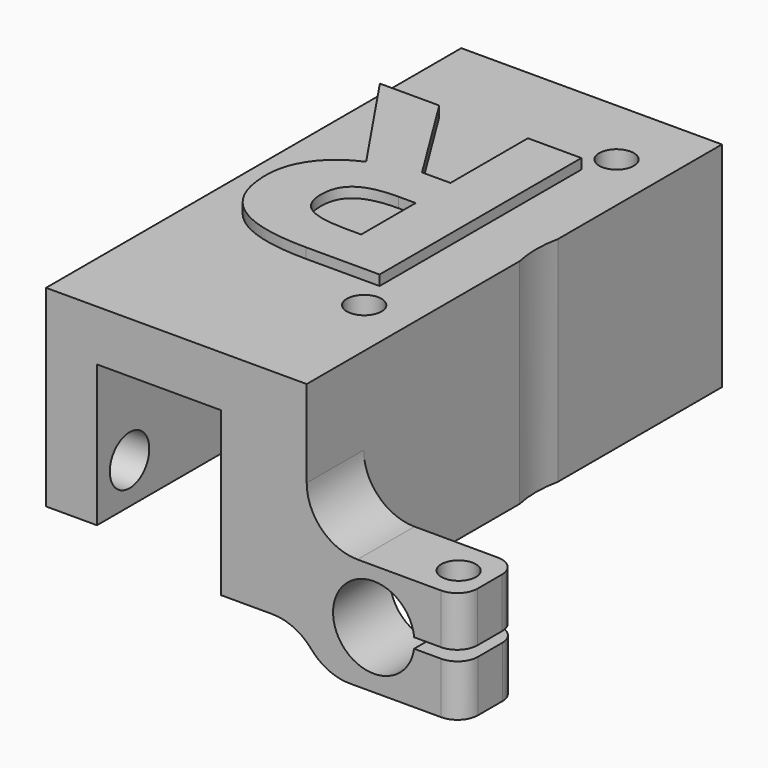
from build123d import *

# Parameters (mm, degrees)
F1_DEPTH      = 7
F2_DEPTH      = 44
F3_R          = 1.7
F3_R_2        = 11
F4_DEPTH      = 21.001
F5_R          = 4
F6_DEPTH      = 10
F7_DEPTH      = 21.001
F8_R          = 1.4
F9_DEPTH      = 11.0207610561
F8_R_2        = 1.7
F10_DEPTH     = 4.9110969969
F11_R         = 5
F12_R         = 5
F13_R         = 5
F14_R         = 2
F15_R         = 2.2
F15_R_2       = 2.4255023423
F16_DEPTH     = 6
F17_TEXT_SIZE = 34.7222222222
F18_DEPTH     = 1


# Not quite as in the source:
# - a feature names something its author has since deleted; it is built from what else it names
# - Text() gives the source's letters only with a copy of the font that has no kerning and outlines rounded to 1/6400 em; it was checked with that copy


with BuildPart() as f1:
    # F0 (on Front) → F1 (new body)
    with BuildSketch(Plane.XZ):
        Polygon((-18.6721007523, 29.8099789735), (-18.6721007523, 10.8925135386), (-13.6721007523, 10.8925135386), (-13.6721007523, 24.8099789735), (-1.4721007523, 24.8099789735), (-1.4721007523, 8.8099789735), (6.9380548998, 8.8099789735), (6.9380548998, 16.2656020473), (6.9380548998, 29.8099789735), align=None)
        Polygon((22.1263195603, 16.2417280634), (6.9380548998, 16.2656020473), (6.9380548998, 8.8099789735), (8.3533044869, 5.2860832236), (22.1553367778, 5.2860832236), (22.1553367778, 10.343908232), (15.4860510706, 10.343908232), (15.4860510706, 11.3388913612), (22.1263195603, 11.3388913612), align=None)
    extrude(amount=F1_DEPTH)

    # F0 (on Front) → F2 (join)
    with BuildSketch(Plane.XZ):
        Polygon((-18.6721007523, 29.8099789735), (-18.6721007523, 10.8925135386), (-13.6721007523, 10.8925135386), (-13.6721007523, 24.8099789735), (-1.4721007523, 24.8099789735), (-1.4721007523, 8.8099789735), (6.9380548998, 8.8099789735), (6.9380548998, 16.2656020473), (6.9380548998, 29.8099789735), align=None)
    extrude(amount=-F2_DEPTH)

    # F3 (on face) → F4 (cut, through all)
    with BuildSketch(Plane(origin=(0, 0, 8.8099789735), x_dir=(1, 0, 0), z_dir=(0, 0, -1))):
        with Locations((2.1850741468, -6)):
            Circle(F3_R)
        with Locations((2.1850741468, -37)):
            Circle(F3_R)
        with Locations((17.6850741468, -21.5)):
            Circle(F3_R_2)
    extrude(amount=-F4_DEPTH, mode=Mode.SUBTRACT)

    # F5 (on face) → F6 (cut)
    with BuildSketch(Plane.XZ.offset(7)):
        with Locations((13.5278992477, 10.8989789735)):
            Circle(F5_R)
    extrude(amount=-F6_DEPTH, mode=Mode.SUBTRACT)

    # F3 (on face) → F7 (cut, through all)
    with BuildSketch(Plane(origin=(0, 0, 8.8099789735), x_dir=(1, 0, 0), z_dir=(0, 0, -1))):
        with Locations((2.1850741468, -6)):
            Circle(F3_R)
        with Locations((2.1850741468, -37)):
            Circle(F3_R)
        with Locations((17.6850741468, -21.5)):
            Circle(F3_R_2)
    extrude(amount=-F7_DEPTH, mode=Mode.SUBTRACT)

    # F8 (on face) → F9 (cut, through all)
    with BuildSketch(Plane(origin=(0.0255844979, 0, 16.2764675551), x_dir=(0.9999987646, 0, -0.0015718685), z_dir=(0.0015718685, 0, 0.9999987646))):
        with Locations((19.1007623654, -3.5767070949)):
            Circle(F8_R)
    extrude(amount=-F9_DEPTH, mode=Mode.SUBTRACT)

    # F8 (on face) → F10 (cut, through all)
    with BuildSketch(Plane(origin=(0.0255844979, 0, 16.2764675551), x_dir=(0.9999987646, 0, -0.0015718685), z_dir=(0.0015718685, 0, 0.9999987646))):
        with Locations((19.1007623654, -3.5767070949)):
            Circle(F8_R_2)
        with Locations((19.1007623654, -3.5767070949)):
            Circle(F8_R, mode=Mode.SUBTRACT)
    extrude(amount=-F10_DEPTH, mode=Mode.SUBTRACT)

    # F11
    f11_edges = [f1.edges().sort_by_distance(p)[0] for p in [
        (6.938055, -3.5, 16.265602),
    ]]
    fillet(f11_edges, radius=F11_R)

    # F12
    f12_edges = [f1.edges().sort_by_distance(p)[0] for p in [
        (6.938055, -3.5, 8.809979),
    ]]
    fillet(f12_edges, radius=F12_R)

    # F13
    f13_edges = [f1.edges().sort_by_distance(p)[0] for p in [
        (8.353304, -3.5, 5.286083),
    ]]
    fillet(f13_edges, radius=F13_R)

    # F14
    f14_edges = [f1.edges().sort_by_distance(p)[0] for p in [
        (22.12632, -7, 13.79031),
        (22.155337, -7, 7.814996),
        (22.12632, 0, 13.79031),
        (22.155337, 0, 7.814996),
    ]]
    fillet(f14_edges, radius=F14_R)

    # F15 (on face) → F16 (cut)
    with BuildSketch(Plane(origin=(-18.6721007523, 0, 0), x_dir=(0, -1, 0), z_dir=(-1, 0, 0))):
        with Locations((-40, 14.8925135386)):
            Circle(F15_R)
        with Locations((3, 14.8925135386)):
            Circle(F15_R_2)
    extrude(amount=-F16_DEPTH, mode=Mode.SUBTRACT)

    # F17 (on face) → F18 (join)
    with BuildSketch(Plane.XY.offset(29.8099789735)):
        with Locations(Location((4.2499912616, 34), (0, 0, 180))):
            Text('R', F17_TEXT_SIZE, font='Open Sans', font_style=FontStyle.BOLD, text_align=(TextAlign.LEFT, TextAlign.BOTTOM))
    extrude(amount=F18_DEPTH)


solid = f1.part
